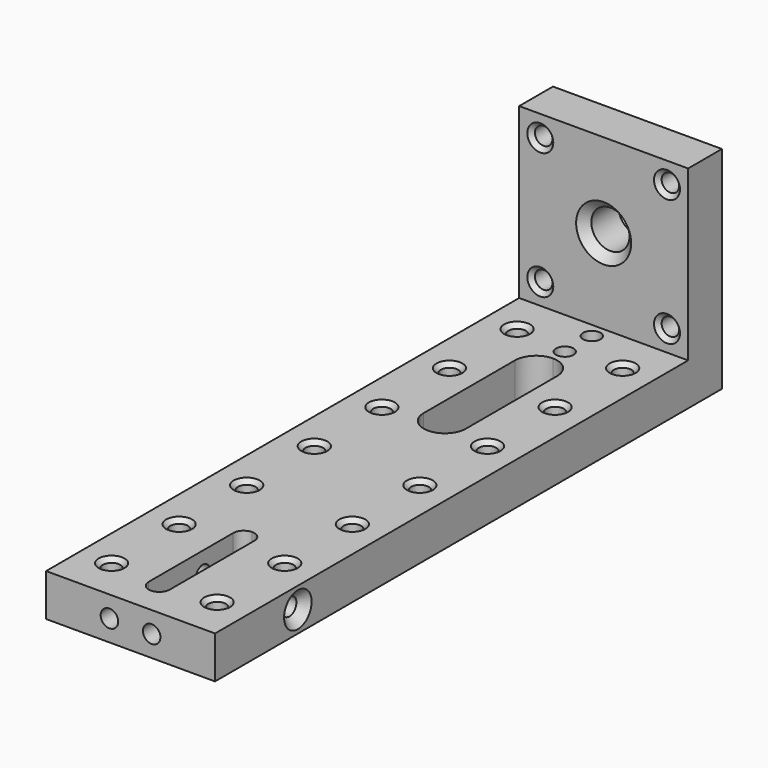
from build123d import *

# Parameters (mm, degrees)
F0_W      = 40
F0_H      = 50
F0_R      = 2.074
F0_R_2    = 4.515
F1_DEPTH  = 10
F2_W      = 40
F2_H      = 10
F3_DEPTH  = 140
F4_SIZE   = 1
F5_SIZE   = 2
F6_W      = 10
F6_H      = 37
F7_DEPTH  = 10
F8_R      = 4.99999
F9_R      = 2.074
F10_DEPTH = 10
F11_R     = 2.074
F12_DEPTH = 10.001
F13_R     = 2.074
F14_DEPTH = 16
F15_SIZE  = 1
F16_SIZE  = 1
F17_W     = 5
F17_H     = 30
F18_DEPTH = 10.001
F19_R     = 2.49999
F20_R     = 2.074
F21_DEPTH = 40.001
F22_SIZE  = 2


# Not quite as in the source:
# - a fillet or chamfer is up to 0.001 mm smaller than in the source, because OpenCascade refuses the exact size


with BuildPart() as f1:
    # F0 (on Front) → F1 (new body)
    with BuildSketch(Plane.XZ):
        with Locations((0, -5)):
            Rectangle(F0_W, F0_H)
        with Locations((-15, -15)):
            Circle(F0_R, mode=Mode.SUBTRACT)
        with Locations((15, -15)):
            Circle(F0_R, mode=Mode.SUBTRACT)
        with Locations((-15, 15)):
            Circle(F0_R, mode=Mode.SUBTRACT)
        Circle(F0_R_2, mode=Mode.SUBTRACT)
        with Locations((15, 15)):
            Circle(F0_R, mode=Mode.SUBTRACT)
    extrude(amount=F1_DEPTH)

    # F2 (on face) → F3 (join)
    with BuildSketch(Plane.XZ.offset(10)):
        with Locations((0, -25)):
            Rectangle(F2_W, F2_H)
    extrude(amount=F3_DEPTH)

    # F4
    f4_edges = [f1.edges().sort_by_distance(p)[0] for p in [
        (-17.074, -10, 15),
        (12.926, -10, 15),
        (12.926, -10, -15),
        (-17.074, -10, -15),
    ]]
    chamfer(f4_edges, length=F4_SIZE)

    # F5
    f5_edges = [f1.edges().sort_by_distance(p)[0] for p in [
        (-4.515, -10, 0),
    ]]
    chamfer(f5_edges, length=F5_SIZE)

    # F6 (on face) → F7 (cut, through all)
    with BuildSketch(Plane.XY.offset(-20)):
        with Locations((0, -43.5)):
            Rectangle(F6_W, F6_H)
    extrude(amount=-F7_DEPTH, mode=Mode.SUBTRACT)

    # F8 (radius 5 in the source; OpenCascade refuses exactly that, so slightly less here)
    f8_edges = [f1.edges().sort_by_distance(p)[0] for p in [
        (5, -62, -25),
        (-5, -62, -25),
        (5, -25, -25),
        (-5, -25, -25),
    ]]
    fillet(f8_edges, radius=F8_R)

    # F9 (on face) → F10 (cut, through all)
    with BuildSketch(Plane.XY.offset(-20)):
        with Locations((-12.5, -140)):
            Circle(F9_R)
        with Locations((-12.5, -120)):
            Circle(F9_R)
        with Locations((-12.5, -100)):
            Circle(F9_R)
        with Locations((-12.5, -80)):
            Circle(F9_R)
        with Locations((-12.5, -60)):
            Circle(F9_R)
        with Locations((12.5, -60)):
            Circle(F9_R)
        with Locations((12.5, -80)):
            Circle(F9_R)
        with Locations((12.5, -100)):
            Circle(F9_R)
        with Locations((12.5, -140)):
            Circle(F9_R)
        with Locations((12.5, -120)):
            Circle(F9_R)
        with Locations((-12.5, -40)):
            Circle(F9_R)
        with Locations((-12.5, -20)):
            Circle(F9_R)
        with Locations((12.5, -40)):
            Circle(F9_R)
        with Locations((12.5, -20)):
            Circle(F9_R)
    extrude(amount=-F10_DEPTH, mode=Mode.SUBTRACT)

    # F11 (on face) → F12 (cut, through all)
    with BuildSketch(Plane.XY.offset(-20)):
        with Locations((0, -13.5)):
            Circle(F11_R)
        with Locations((0, -21.5)):
            Circle(F11_R)
    extrude(amount=-F12_DEPTH, mode=Mode.SUBTRACT)

    # F13 (on face) → F14 (cut)
    with BuildSketch(Plane.XZ.offset(150)):
        with Locations((-5, -25)):
            Circle(F13_R)
        with Locations((5, -25)):
            Circle(F13_R)
    extrude(amount=-F14_DEPTH, mode=Mode.SUBTRACT)

    # F15
    f15_edges = [f1.edges().sort_by_distance(p)[0] for p in [
        (-2.074, -21.5, -30),
        (-2.074, -13.5, -30),
    ]]
    chamfer(f15_edges, length=F15_SIZE)

    # F16
    f16_edges = [f1.edges().sort_by_distance(p)[0] for p in [
        (-14.574, -140, -20),
        (10.426, -140, -20),
        (10.426, -120, -20),
        (-14.574, -120, -20),
        (10.426, -100, -20),
        (-14.574, -100, -20),
        (10.426, -80, -20),
        (-14.574, -80, -20),
        (10.426, -60, -20),
        (-14.574, -60, -20),
        (-14.574, -40, -20),
        (10.426, -40, -20),
        (-10.426, -20, -25),
        (-14.574, -20, -20),
        (-14.574, -20, -30),
        (14.574, -20, -25),
        (10.426, -20, -20),
        (10.426, -20, -30),
    ]]
    chamfer(f16_edges, length=F16_SIZE)

    # F17 (on face) → F18 (cut, through all)
    with BuildSketch(Plane.XY.offset(-20)):
        with Locations((0, -129)):
            Rectangle(F17_W, F17_H)
    extrude(amount=-F18_DEPTH, mode=Mode.SUBTRACT)

    # F19 (radius 2.5 in the source; OpenCascade refuses exactly that, so slightly less here)
    f19_edges = [f1.edges().sort_by_distance(p)[0] for p in [
        (-2.5, -144, -25),
        (2.5, -144, -25),
        (-2.5, -114, -25),
        (2.5, -114, -25),
    ]]
    fillet(f19_edges, radius=F19_R)

    # F20 (on face) → F21 (cut, through all)
    with BuildSketch(Plane(origin=(-20, 0, 0), x_dir=(0, -1, 0), z_dir=(-1, 0, 0))):
        with Locations((125.5, -25)):
            Circle(F20_R)
    extrude(amount=-F21_DEPTH, mode=Mode.SUBTRACT)

    # F22
    f22_edges = [f1.edges().sort_by_distance(p)[0] for p in [
        (-20, -123.426, -25),
        (20, -123.426, -25),
    ]]
    chamfer(f22_edges, length=F22_SIZE)


solid = f1.part
